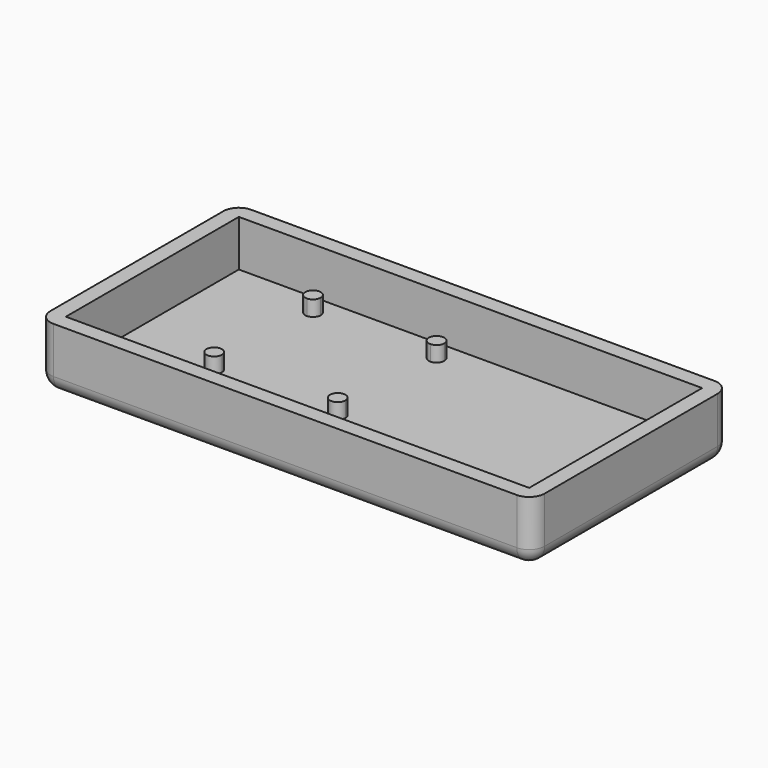
from build123d import *

# Parameters (mm, degrees)
F0_W     = 203.2
F0_H     = 101.6
F1_DEPTH = 25.4
F2_R     = 6.35
F3_T     = 6.35
F5_DEPTH = 6.35


# Not quite as in the source:
# - a shell that OpenCascade refuses in one call is made with other operations: the cavity is built on its own and cut out


with BuildPart() as f1:
    # F0 (on Top) → F1 (new body)
    with BuildSketch(Plane.XY):
        with Locations((101.6, 50.8)):
            Rectangle(F0_W, F0_H)
    extrude(amount=F1_DEPTH)

    # F2
    f2_edges = [f1.edges().sort_by_distance(p)[0] for p in [
        (0, 0, 12.7),
        (203.2, 0, 12.7),
        (0, 101.6, 12.7),
        (203.2, 101.6, 12.7),
        (101.6, 101.6, 0),
        (0, 50.8, 0),
        (101.6, 0, 0),
        (203.2, 50.8, 0),
    ]]
    fillet(f2_edges, radius=F2_R)

    # F3: shell of thickness 6.35, made by hand


with BuildPart() as f3_core1:
    # F3_t2: copy of F1
    add(f1.part)

    # the walls: a layer under each face that stays
    f3_faces = [f3_core1.faces().sort_by_distance(p)[0] for p in [
        (0, 50.8, 15.875),
        (101.6, 101.6, 15.875),
        (101.6, 0, 15.875),
        (203.2, 50.8, 15.875),
        (101.6, 50.8, 0),
    ]]
    thicken(f3_faces, amount=-F3_T, mode=Mode.SUBTRACT)


with BuildPart() as f1_1:
    add(f1.part)

    # what is left inside the walls is the cavity
    f3_cavity = [f3_core1.part.solids().sort_by_distance(p)[0] for p in [
        (101.6, 35.983333, 25.3365),
    ]]
    add(f3_cavity, mode=Mode.SUBTRACT)

    # F4 (on face) → F5 (join)
    with BuildSketch(Plane.XY.offset(6.35)):
        with BuildLine():
            Line((43.5933910498, 86.815246595), (46.7683910498, 86.815246595))
            ThreePointArc((46.7683910498, 86.815246595), (41.3483270196, 89.0603106253), (43.5933910498, 83.640246595))
            Line((43.5933910498, 83.640246595), (43.5933910498, 86.815246595))
        make_face()
        with BuildLine():
            ThreePointArc((43.5933910498, 83.640246595), (45.8384550801, 84.5701825647), (46.7683910498, 86.815246595))
            Line((46.7683910498, 86.815246595), (43.5933910498, 86.815246595))
            Line((43.5933910498, 86.815246595), (43.5933910498, 83.640246595))
        make_face()
        with BuildLine():
            ThreePointArc((97.5683910498, 86.815246595), (94.3933910498, 89.990246595), (91.2183910498, 86.815246595))
            Line((91.2183910498, 86.815246595), (94.3933910498, 86.815246595))
            Line((94.3933910498, 86.815246595), (94.3933910498, 83.640246595))
            ThreePointArc((94.3933910498, 83.640246595), (96.6384550801, 84.5701825647), (97.5683910498, 86.815246595))
        make_face()
        with BuildLine():
            Line((94.3933910498, 86.815246595), (91.2183910498, 86.815246595))
            ThreePointArc((91.2183910498, 86.815246595), (92.1483270196, 84.5701825647), (94.3933910498, 83.640246595))
            Line((94.3933910498, 83.640246595), (94.3933910498, 86.815246595))
        make_face()
        with BuildLine():
            Line((94.3933910498, 36.015246595), (94.3933910498, 39.190246595))
            ThreePointArc((94.3933910498, 39.190246595), (92.1483270196, 38.2603106253), (91.2183910498, 36.015246595))
            Line((91.2183910498, 36.015246595), (94.3933910498, 36.015246595))
        make_face()
        with BuildLine():
            ThreePointArc((46.7683910498, 36.015246595), (45.8384550801, 38.2603106253), (43.5933910498, 39.190246595))
            Line((43.5933910498, 39.190246595), (43.5933910498, 36.015246595))
            Line((43.5933910498, 36.015246595), (46.7683910498, 36.015246595))
        make_face()
        with BuildLine():
            Line((43.5933910498, 36.015246595), (43.5933910498, 39.190246595))
            ThreePointArc((43.5933910498, 39.190246595), (41.3483270196, 33.7701825647), (46.7683910498, 36.015246595))
            Line((46.7683910498, 36.015246595), (43.5933910498, 36.015246595))
        make_face()
        with BuildLine():
            ThreePointArc((97.5683910498, 36.015246595), (96.6384550801, 38.2603106253), (94.3933910498, 39.190246595))
            Line((94.3933910498, 39.190246595), (94.3933910498, 36.015246595))
            Line((94.3933910498, 36.015246595), (91.2183910498, 36.015246595))
            ThreePointArc((91.2183910498, 36.015246595), (94.3933910498, 32.840246595), (97.5683910498, 36.015246595))
        make_face()
    extrude(amount=F5_DEPTH)


solid = f1_1.part
